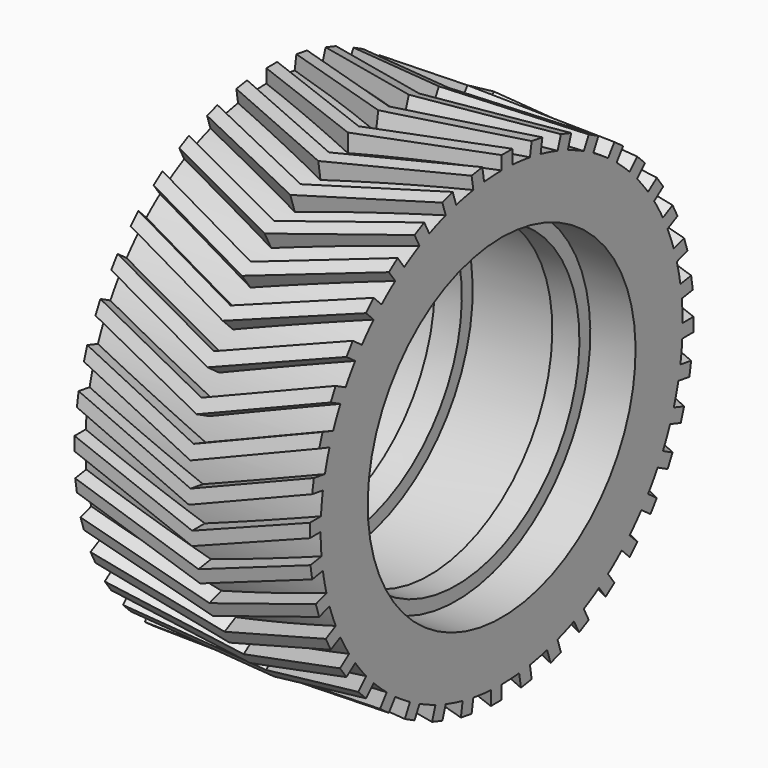
from build123d import *

# Parameters (mm, degrees)
F3_START = 23.5
F3_DEPTH = 3
F4_COUNT = 40


with BuildPart() as f1:
    # F0 (on Front) → F1 (revolve)
    with BuildSketch(Plane.XZ):
        Polygon((-5, 17), (-5, 18.5), (5, 18.5), (5, 17), (8, 17), (8, 18.5), (13, 18.5), (13, 25), (-13, 25), (-13, 18.5), (-8, 18.5), (-8, 17), align=None)
    revolve(axis=Axis((0, 0, 0), (1, 0, 0)))

    # F2 (on Top) → F3 (join)
    with BuildSketch(Plane.XY.offset(F3_START)):
        Polygon((-13, 1.5), (-13, 0), (0, -5), (13, 0), (13, 1.5), (0, -3.5), align=None)
    extrude(amount=F3_DEPTH)

    # F4: F1 ×40 about axis
    f4_axis = Axis((0, 0, 0), (1, 0, 0))


with BuildPart() as f1_1:
    add(f1.part)
    for i in range(1, F4_COUNT):
        add(f1.part.rotate(f4_axis, i * 360 / F4_COUNT))


solid = f1_1.part
